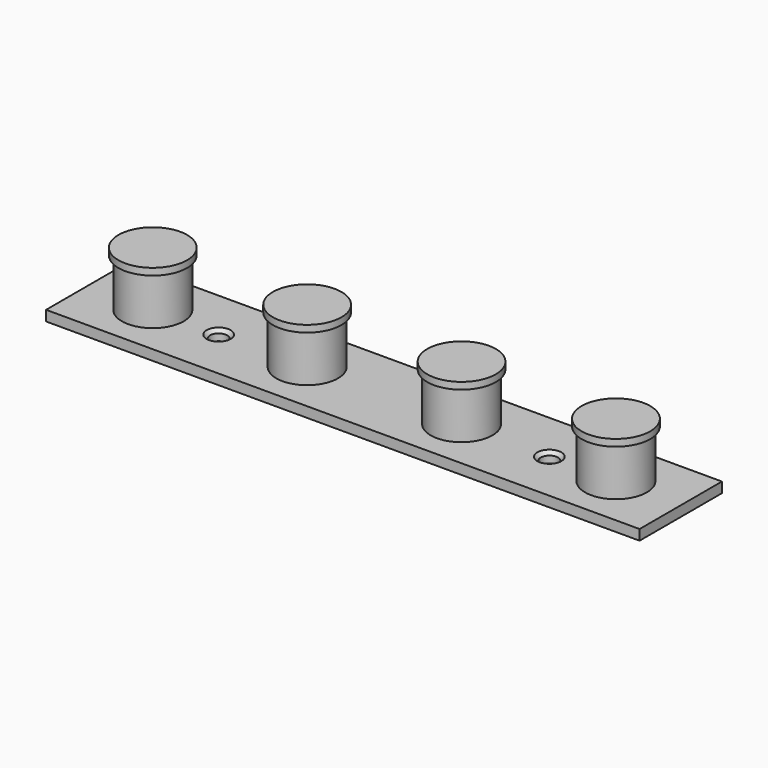
from build123d import *

# Parameters (mm, degrees)
F0_W     = 173
F0_H     = 30
F1_DEPTH = 3
F2_R     = 9
F3_DEPTH = 15
F4_R     = 2.5
F5_DEPTH = 25
F6_SIZE  = 1
F7_R     = 10
F7_R_2   = 9
F8_DEPTH = 1


with BuildPart() as f1:
    # F0 (on Top) → F1 (new body)
    with BuildSketch(Plane.XY):
        Rectangle(F0_W, F0_H)
    extrude(amount=-F1_DEPTH)

    # F2 (on face) → F3 (join)
    with BuildSketch(Plane.XY):
        with Locations((-67.5, 0.1318904841)):
            Circle(F2_R)
        with Locations((-22.5, 0.1318904841)):
            Circle(F2_R)
        with Locations((22.5, 0.1318904841)):
            Circle(F2_R)
        with Locations((67.5, 0.1318904841)):
            Circle(F2_R)
    extrude(amount=F3_DEPTH)

    # F4 (on face) → F5 (cut)
    with BuildSketch(Plane.XY):
        with Locations((-48.203933984, 0)):
            Circle(F4_R)
        with Locations((48.203933984, 0)):
            Circle(F4_R)
    extrude(amount=-F5_DEPTH, mode=Mode.SUBTRACT)

    # F6
    f6_edges = [f1.edges().sort_by_distance(p)[0] for p in [
        (-50.703934, 0, 0),
        (45.703934, 0, 0),
    ]]
    chamfer(f6_edges, length=F6_SIZE)

    # F7 (on face) → F8 (join, symmetric)
    with BuildSketch(Plane.XY.offset(15)):
        with Locations((-67.5, 0.1318904841)):
            Circle(F7_R)
        with Locations((-67.5, 0.1318904841)):
            Circle(F7_R_2, mode=Mode.SUBTRACT)
        with Locations((-22.5, 0.1318904841)):
            Circle(F7_R)
        with Locations((22.5, 0.1318904841)):
            Circle(F7_R)
        with Locations((67.5, 0.1318904841)):
            Circle(F7_R)
        with Locations((-67.5, 0.1318904841)):
            Circle(F7_R_2)
    extrude(amount=F8_DEPTH, both=True)


solid = f1.part
